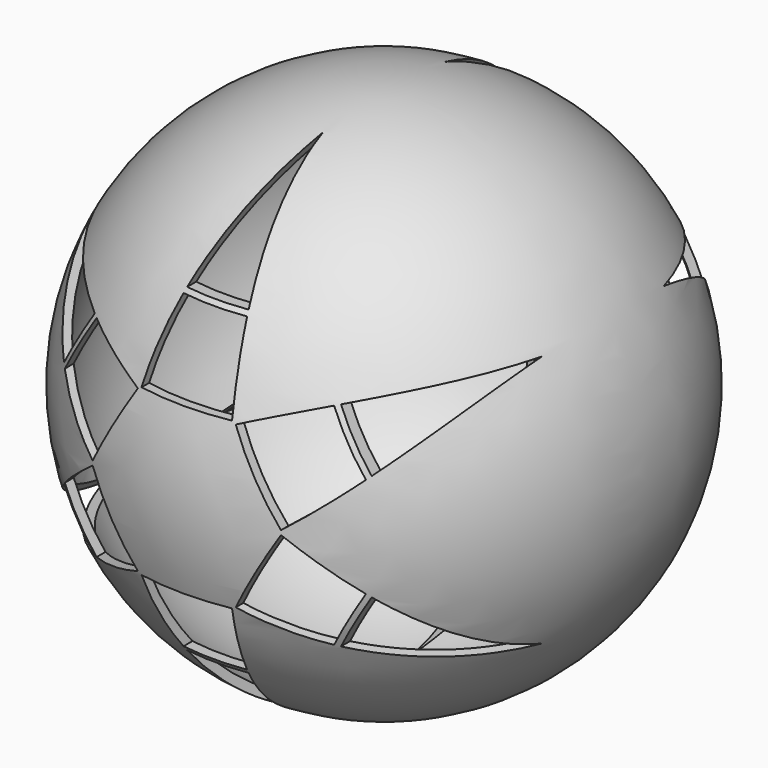
from build123d import *

# Parameters (mm, degrees)
F4_DEPTH        = 330.2
F4_COPIES_COUNT = 3
F4_COPIES_ANGLE = 120


# Not quite as in the source:
# - a pattern or mirror of a feature is missing from the dataset's text; its kind, count and spacing are read off the source's solid


with BuildPart() as f1:
    # F0 (on Front) → F1 (revolve)
    with BuildSketch(Plane.XZ):
        with BuildLine():
            Line((0, -147.32), (0, -152.4))
            ThreePointArc((0, -152.4), (152.4, 0), (0, 152.4))
            Line((0, 152.4), (0, 147.32))
            ThreePointArc((0, 147.32), (147.32, 0), (0, -147.32))
        make_face()
    revolve(axis=Axis((0, 0, 0), (0, 0, -1)))

    # F3 (on offset) → F4 (cut)
    with BuildSketch(Plane.XZ.offset(152.4)):
        with BuildLine():
            Line((-17.7398536878, 92.3459759731), (17.7398536878, 92.3459759731))
            ThreePointArc((17.7398536878, 92.3459759731), (9.8655778035, 119.4568227482), (0, 145.9081480113))
            ThreePointArc((0, 145.9081480113), (-9.8655778035, 119.4568227482), (-17.7398536878, 92.3459759731))
        make_face()
        with BuildLine():
            ThreePointArc((26.1251415889, 47.7141484516), (22.839247984, 68.8693933573), (18.3670011022, 89.8059759731))
            Line((18.3670011022, 89.8059759731), (-18.3670011022, 89.8059759731))
            ThreePointArc((-18.3670011022, 89.8059759731), (-22.839247984, 68.8693933573), (-26.1251415889, 47.7141484516))
            Line((-26.1251415889, 47.7141484516), (26.1251415889, 47.7141484516))
        make_face()
        with BuildLine():
            ThreePointArc((18.3670011022, -89.8059759731), (22.839247984, -68.8693933573), (26.1251415889, -47.7141484516))
            Line((26.1251415889, -47.7141484516), (-26.1251415889, -47.7141484516))
            ThreePointArc((-26.1251415889, -47.7141484516), (-22.839247984, -68.8693933573), (-18.3670011022, -89.8059759731))
            Line((-18.3670011022, -89.8059759731), (18.3670011022, -89.8059759731))
        make_face()
        with BuildLine():
            ThreePointArc((-17.7398536878, -92.3459759731), (-9.8655778035, -119.4568227482), (0, -145.9081480113))
            ThreePointArc((0, -145.9081480113), (9.8655778035, -119.4568227482), (17.7398536878, -92.3459759731))
            Line((17.7398536878, -92.3459759731), (-17.7398536878, -92.3459759731))
        make_face()
    f4 = extrude(amount=-F4_DEPTH, mode=Mode.SUBTRACT)

    # F4_copies: F4 ×3 about axis
    f4_copies_axis = Axis((0, 0, 0), (0, 1, 0))
    for i in range(1, F4_COPIES_COUNT):
        add(f4.rotate(f4_copies_axis, i * F4_COPIES_ANGLE / (F4_COPIES_COUNT - 1)), mode=Mode.SUBTRACT)


solid = f1.part
